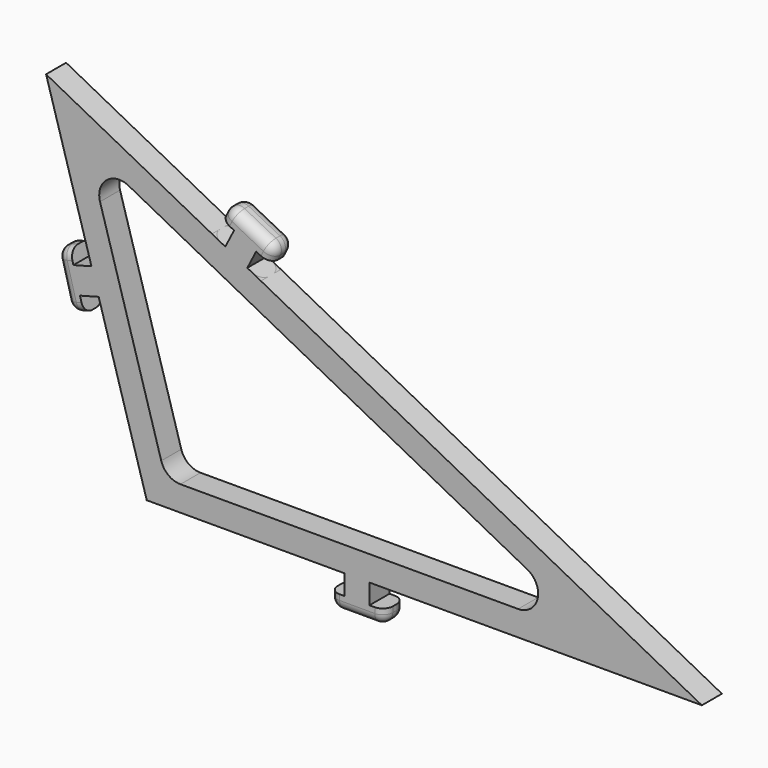
from build123d import *

# Parameters (mm, degrees)
F1_DEPTH      = 6.35
F2_R          = 5.08
F4_DEPTH      = 6.35
F5_R          = 2.54
F6_R          = 2.54
F7_R          = 2.54
F8_R          = 2.54
F10_DEPTH     = 6.35
F11_R         = 2.54
F12_R         = 2.54
F13_T1_DEPTH  = 8.9083831143
F13_T3_DEPTH  = 1.27
F13_T6_ANGLE  = 90
F13_T8_ANGLE  = 90
F13_T10_ANGLE = 90
F13_T12_ANGLE = 90
F15_DEPTH     = 6.35
F16_R         = 2.54
F17_T1_DEPTH  = 1.27
F17_T4_ANGLE  = 90
F17_T6_ANGLE  = 90
F17_T10_DEPTH = 7.7319413884
F17_T15_DEPTH = 7.7319413884
F18_T1_DEPTH  = 1.27
F18_T4_ANGLE  = 90
F18_T8_DEPTH  = 7.7319413884
F18_T13_DEPTH = 7.7319413884
F18_T16_ANGLE = 90


# Not quite as in the source:
# - a fillet or chamfer that OpenCascade refuses, or shapes differently, is made with other operations: its cross-section is extruded or revolved along the edge and cut away or added


with BuildPart() as f1:
    # F0 (on Front) → F1 (new body)
    with BuildSketch(Plane.XZ):
        Polygon((-140.7776176929, 0), (0, 0), (-166.3033664227, 86.8016779423), align=None)
        Polygon((-136.0260884312, 6.35), (-155.9960301785, 74.2588582448), (-25.8894239036, 6.35), align=None, mode=Mode.SUBTRACT)
    extrude(amount=F1_DEPTH)

    # F2
    f2_edges = [f1.edges().sort_by_distance(p)[0] for p in [
        (-155.99603, -3.175, 74.258858),
        (-25.889424, -3.175, 6.35),
        (-136.026088, -3.175, 6.35),
    ]]
    fillet(f2_edges, radius=F2_R)

    # F3 (on Front) → F4 (join)
    with BuildSketch(Plane.XZ):
        Polygon((-84.2989161611, 0), (-90.5948132277, 0), (-90.5948132277, -5.0825621001), (-94.4040864706, -5.0825621001), (-94.4040864706, -9.0045034885), (-80.4157033563, -9.0045034885), (-80.4157033563, -5.0825621001), (-84.2989161611, -5.0825621001), align=None)
    extrude(amount=F4_DEPTH)

    # F5
    f5_edges = [f1.edges().sort_by_distance(p)[0] for p in [
        (-80.415703, 0, -7.043533),
    ]]
    fillet(f5_edges, radius=F5_R)

    # F6
    f6_edges = [f1.edges().sort_by_distance(p)[0] for p in [
        (-94.404086, 0, -7.043533),
    ]]
    fillet(f6_edges, radius=F6_R)

    # F7
    f7_edges = [f1.edges().sort_by_distance(p)[0] for p in [
        (-94.404086, -6.35, -7.043533),
        (-80.415703, -6.35, -7.043533),
    ]]
    fillet(f7_edges, radius=F7_R)

    # F8
    f8_edges = [f1.edges().sort_by_distance(p)[0] for p in [
        (-87.409895, -6.35, -9.004503),
        (-87.409895, 0, -9.004503),
    ]]
    fillet(f8_edges, radius=F8_R)

    # F9 (on face) → F10 (join)
    with BuildSketch(Plane(origin=(0, 0, 0), x_dir=(-1, 0, 0), z_dir=(0, 1, 0))):
        Polygon((154.6036799573, 47.7280417937), (152.9238455726, 41.4588145216), (152.9660739724, 41.4474994559), (154.7977033408, 47.6760533848), align=None)
        Polygon((154.7977033408, 47.6760533848), (152.9660739724, 41.4474994559), (157.7012996051, 40.1786995717), (156.6624483483, 36.3016538997), (160.4507528245, 35.2865807746), (164.0712127847, 48.7983212928), (160.2829083085, 49.8133944179), (159.3811339898, 46.4479268438), align=None)
    extrude(amount=-F10_DEPTH)

    # F11
    f11_edges = [f1.edges().sort_by_distance(p)[0] for p in [
        (-162.177061, -6.35, 49.305858),
        (-158.556601, -6.35, 35.794117),
    ]]
    fillet(f11_edges, radius=F11_R)

    # F12
    f12_edges = [f1.edges().sort_by_distance(p)[0] for p in [
        (-162.177061, 0, 49.305858),
        (-158.556601, 0, 35.794117),
    ]]
    fillet(f12_edges, radius=F12_R)

    # F13: fillet of radius 2.54 on 6 edges, made by hand

    # F13_s2 → F13_t1 (cut)
    with BuildSketch(Plane(origin=(-20.2272079793, 0, 75.488967874), x_dir=(0, 1, 0), z_dir=(-0.2588190451, 0, 0.9659258263))):
        with BuildLine():
            ThreePointArc((0, 143.3106868597), (-0.7439487758, 145.1067380839), (-2.54, 145.8506868597))
            Line((-2.54, 145.8506868597), (0, 145.8506868597))
            Line((0, 145.8506868597), (0, 143.3106868597))
        make_face()
        with BuildLine():
            ThreePointArc((-6.35, 143.3106868597), (-5.6060512242, 145.1067380839), (-3.81, 145.8506868597))
            Line((-3.81, 145.8506868597), (-6.35, 145.8506868597))
            Line((-6.35, 145.8506868597), (-6.35, 143.3106868597))
        make_face()
    extrude(amount=F13_T1_DEPTH, mode=Mode.SUBTRACT)

    # F13_s4 → F13_t3 (cut)
    with BuildSketch(Plane.XZ.offset(2.54)):
        with BuildLine():
            ThreePointArc((-161.1081531991, 37.7400323734), (-159.9247016003, 36.1977282224), (-157.9973012258, 35.9439811492))
            Line((-157.9973012258, 35.9439811492), (-160.4507528245, 35.2865807746))
            Line((-160.4507528245, 35.2865807746), (-161.1081531991, 37.7400323734))
        make_face()
        with BuildLine():
            ThreePointArc((-161.617761186, 49.4557216674), (-163.160065337, 48.2722700686), (-163.4138124102, 46.344869694))
            Line((-163.4138124102, 46.344869694), (-164.0712127847, 48.7983212928))
            Line((-164.0712127847, 48.7983212928), (-161.617761186, 49.4557216674))
        make_face()
    extrude(amount=F13_T3_DEPTH, mode=Mode.SUBTRACT)

    # F13_s5 → F13_t6 (revolve, cut)
    with BuildSketch(Plane.XZ.offset(2.54)):
        with BuildLine():
            ThreePointArc((-161.617761186, 49.4557216674), (-163.160065337, 48.2722700686), (-163.4138124102, 46.344869694))
            Line((-163.4138124102, 46.344869694), (-164.0712127847, 48.7983212928))
            Line((-164.0712127847, 48.7983212928), (-161.617761186, 49.4557216674))
        make_face()
    revolve(axis=Axis((-163.4138124102, -2.54, 46.344869694), (-0.9659258263, 0, -0.2588190451)), revolution_arc=F13_T6_ANGLE, mode=Mode.SUBTRACT)

    # F13_s7 → F13_t8 (revolve, cut)
    with BuildSketch(Plane(origin=(-22.5328671904, 0, 84.0938051946), x_dir=(0, 1, 0), z_dir=(0.2588190451, 0, -0.9659258263))):
        with BuildLine():
            ThreePointArc((-6.35, -143.3106868597), (-5.6060512242, -145.1067380839), (-3.81, -145.8506868597))
            Line((-3.81, -145.8506868597), (-6.35, -145.8506868597))
            Line((-6.35, -145.8506868597), (-6.35, -143.3106868597))
        make_face()
    revolve(axis=Axis((-163.4138124102, -3.81, 46.344869694), (-0.9659258263, 0, -0.2588190451)), revolution_arc=F13_T8_ANGLE, mode=Mode.SUBTRACT)

    # F13_s9 → F13_t10 (revolve, cut)
    with BuildSketch(Plane(origin=(-20.2272079793, 0, 75.488967874), x_dir=(0, 1, 0), z_dir=(-0.2588190451, 0, 0.9659258263))):
        with BuildLine():
            ThreePointArc((-3.81, 145.8506868597), (-5.6060512242, 145.1067380839), (-6.35, 143.3106868597))
            Line((-6.35, 143.3106868597), (-6.35, 145.8506868597))
            Line((-6.35, 145.8506868597), (-3.81, 145.8506868597))
        make_face()
    revolve(axis=Axis((-161.1081531991, -3.81, 37.7400323734), (0.9659258263, 0, 0.2588190451)), revolution_arc=F13_T10_ANGLE, mode=Mode.SUBTRACT)

    # F13_s11 → F13_t12 (revolve, cut)
    with BuildSketch(Plane(origin=(-20.2272079793, 0, 75.488967874), x_dir=(0, 1, 0), z_dir=(-0.2588190451, 0, 0.9659258263))):
        with BuildLine():
            ThreePointArc((-2.54, 145.8506868597), (-0.7439487758, 145.1067380839), (0, 143.3106868597))
            Line((0, 143.3106868597), (0, 145.8506868597))
            Line((0, 145.8506868597), (-2.54, 145.8506868597))
        make_face()
    revolve(axis=Axis((-161.1081531991, -2.54, 37.7400323734), (-0.9659258263, 0, -0.2588190451)), revolution_arc=F13_T12_ANGLE, mode=Mode.SUBTRACT)

    # F14 (on face) → F15 (join)
    with BuildSketch(Plane(origin=(0, 0, 0), x_dir=(-1, 0, 0), z_dir=(0, 1, 0))):
        Polygon((115.2743030785, 60.1671700704), (120.8559281551, 63.0804870568), (118.6355388683, 67.435692909), (122.0292159852, 69.1658715892), (120.2478632331, 72.6599246264), (107.7856289299, 66.3063761433), (109.5669816821, 62.8123231061), (113.026531469, 64.5760852667), align=None)
    extrude(amount=-F15_DEPTH)

    # F16
    f16_edges = [f1.edges().sort_by_distance(p)[0] for p in [
        (-114.016746, -6.35, 69.48315),
        (-114.016746, 0, 69.48315),
    ]]
    fillet(f16_edges, radius=F16_R)

    # F17: fillet of radius 2.54 on 4 edges, made by hand

    # F17_s2 → F17_t1 (cut)
    with BuildSketch(Plane.XZ.offset(2.54)):
        with BuildLine():
            ThreePointArc((-121.4015357494, 70.3970415704), (-119.9229829878, 71.6592386675), (-117.9849801771, 71.50625211))
            Line((-117.9849801771, 71.50625211), (-120.2478632331, 72.6599246264))
            Line((-120.2478632331, 72.6599246264), (-121.4015357494, 70.3970415704))
        make_face()
    extrude(amount=F17_T1_DEPTH, mode=Mode.SUBTRACT)

    # F17_s3 → F17_t4 (revolve, cut)
    with BuildSketch(Plane(origin=(3.4409642411, 0, 6.7493153968), x_dir=(0, 1, 0), z_dir=(-0.4542017781, 0, -0.8908988409))):
        with BuildLine():
            ThreePointArc((0, -137.5909489404), (-0.7439487758, -139.3870001646), (-2.54, -140.1309489404))
            Line((-2.54, -140.1309489404), (0, -140.1309489404))
            Line((0, -140.1309489404), (0, -137.5909489404))
        make_face()
    revolve(axis=Axis((-121.4015357494, -2.54, 70.3970415704), (0.8908988409, 0, -0.4542017781)), revolution_arc=F17_T4_ANGLE, mode=Mode.SUBTRACT)

    # F17_s5 → F17_t6 (revolve, cut)
    with BuildSketch(Plane(origin=(3.4409642411, 0, 6.7493153968), x_dir=(0, 1, 0), z_dir=(-0.4542017781, 0, -0.8908988409))):
        with BuildLine():
            ThreePointArc((-3.81, -140.1309489404), (-5.6060512242, -139.3870001646), (-6.35, -137.5909489404))
            Line((-6.35, -137.5909489404), (-6.35, -140.1309489404))
            Line((-6.35, -140.1309489404), (-3.81, -140.1309489404))
        make_face()
    revolve(axis=Axis((-121.4015357494, -3.81, 70.3970415704), (-0.8908988409, 0, 0.4542017781)), revolution_arc=F17_T6_ANGLE, mode=Mode.SUBTRACT)


with BuildPart() as f17_tool8:
    # F17_s9 → F17_t10 (new body)
    with BuildSketch(Plane(origin=(-0.0708972856, 0, -0.1390622243), x_dir=(0, 1, 0), z_dir=(0.4542017781, 0, 0.8908988409))):
        with BuildLine():
            ThreePointArc((-3.81, 140.1309489404), (-5.6060512242, 139.3870001646), (-6.35, 137.5909489404))
            Line((-6.35, 137.5909489404), (-6.35, 140.1309489404))
            Line((-6.35, 140.1309489404), (-3.81, 140.1309489404))
        make_face()
    extrude(amount=F17_T10_DEPTH)

    split(bisect_by=Plane(origin=(0, 0, 0), x_dir=(0, 1, 0), z_dir=(0.4627114138, 0, 0.8865089664)), keep=Keep.TOP)


with BuildPart() as f1_1:
    add(f1.part)

    # F17_t7: cut F17_tool8
    add(f17_tool8.part, mode=Mode.SUBTRACT)


with BuildPart() as f17_tool13:
    # F17_s14 → F17_t15 (new body)
    with BuildSketch(Plane(origin=(-0.0708972856, 0, -0.1390622243), x_dir=(0, 1, 0), z_dir=(0.4542017781, 0, 0.8908988409))):
        with BuildLine():
            ThreePointArc((0, 137.5909489404), (-0.7439487758, 139.3870001646), (-2.54, 140.1309489404))
            Line((-2.54, 140.1309489404), (0, 140.1309489404))
            Line((0, 140.1309489404), (0, 137.5909489404))
        make_face()
    extrude(amount=F17_T15_DEPTH)

    split(bisect_by=Plane(origin=(0, 0, 0), x_dir=(0, 1, 0), z_dir=(0.4627114138, 0, 0.8865089664)), keep=Keep.TOP)


with BuildPart() as f1_2:
    add(f1_1.part)

    # F17_t12: cut F17_tool13
    add(f17_tool13.part, mode=Mode.SUBTRACT)

    # F18: fillet of radius 2.54 on 5 edges, made by hand

    # F18_s2 → F18_t1 (cut)
    with BuildSketch(Plane.XZ.offset(2.54)):
        with BuildLine():
            ThreePointArc((-110.0485119859, 67.4600486596), (-108.7863148888, 65.981495898), (-108.9393014463, 64.0434930873))
            Line((-108.9393014463, 64.0434930873), (-107.7856289299, 66.3063761433))
            Line((-107.7856289299, 66.3063761433), (-110.0485119859, 67.4600486596))
        make_face()
    extrude(amount=F18_T1_DEPTH, mode=Mode.SUBTRACT)

    # F18_s3 → F18_t4 (revolve, cut)
    with BuildSketch(Plane(origin=(3.4409642411, 0, 6.7493153968), x_dir=(0, 1, 0), z_dir=(-0.4542017781, 0, -0.8908988409))):
        with BuildLine():
            ThreePointArc((0, -128.6825658261), (-0.7439487758, -126.8865146019), (-2.54, -126.1425658261))
            Line((-2.54, -126.1425658261), (0, -126.1425658261))
            Line((0, -126.1425658261), (0, -128.6825658261))
        make_face()
    revolve(axis=Axis((-108.9393014463, -2.54, 64.0434930873), (0.8908988409, 0, -0.4542017781)), revolution_arc=F18_T4_ANGLE, mode=Mode.SUBTRACT)


with BuildPart() as f18_tool6:
    # F18_s7 → F18_t8 (new body)
    with BuildSketch(Plane(origin=(3.4409642411, 0, 6.7493153968), x_dir=(0, 1, 0), z_dir=(-0.4542017781, 0, -0.8908988409))):
        with BuildLine():
            ThreePointArc((0, -128.6825658261), (-0.7439487758, -126.8865146019), (-2.54, -126.1425658261))
            Line((-2.54, -126.1425658261), (0, -126.1425658261))
            Line((0, -126.1425658261), (0, -128.6825658261))
        make_face()
    extrude(amount=F18_T8_DEPTH)

    split(bisect_by=Plane(origin=(0, 0, 0), x_dir=(0, 1, 0), z_dir=(0.4627114138, 0, 0.8865089664)), keep=Keep.TOP)


with BuildPart() as f1_3:
    add(f1_2.part)

    # F18_t5: cut F18_tool6
    add(f18_tool6.part, mode=Mode.SUBTRACT)


with BuildPart() as f18_tool11:
    # F18_s12 → F18_t13 (new body)
    with BuildSketch(Plane(origin=(3.4409642411, 0, 6.7493153968), x_dir=(0, 1, 0), z_dir=(-0.4542017781, 0, -0.8908988409))):
        with BuildLine():
            ThreePointArc((-6.35, -128.6825658261), (-5.6060512242, -126.8865146019), (-3.81, -126.1425658261))
            Line((-3.81, -126.1425658261), (-6.35, -126.1425658261))
            Line((-6.35, -126.1425658261), (-6.35, -128.6825658261))
        make_face()
    extrude(amount=F18_T13_DEPTH)

    split(bisect_by=Plane(origin=(0, 0, 0), x_dir=(0, 1, 0), z_dir=(0.4627114138, 0, 0.8865089664)), keep=Keep.TOP)


with BuildPart() as f1_4:
    add(f1_3.part)

    # F18_t10: cut F18_tool11
    add(f18_tool11.part, mode=Mode.SUBTRACT)

    # F18_s15 → F18_t16 (revolve, cut)
    with BuildSketch(Plane(origin=(3.4409642411, 0, 6.7493153968), x_dir=(0, 1, 0), z_dir=(-0.4542017781, 0, -0.8908988409))):
        with BuildLine():
            ThreePointArc((-6.35, -128.6825658261), (-5.6060512242, -126.8865146019), (-3.81, -126.1425658261))
            Line((-3.81, -126.1425658261), (-6.35, -126.1425658261))
            Line((-6.35, -126.1425658261), (-6.35, -128.6825658261))
        make_face()
    revolve(axis=Axis((-108.9393014463, -3.81, 64.0434930873), (-0.8908988409, 0, 0.4542017781)), revolution_arc=F18_T16_ANGLE, mode=Mode.SUBTRACT)


solid = f1_4.part
